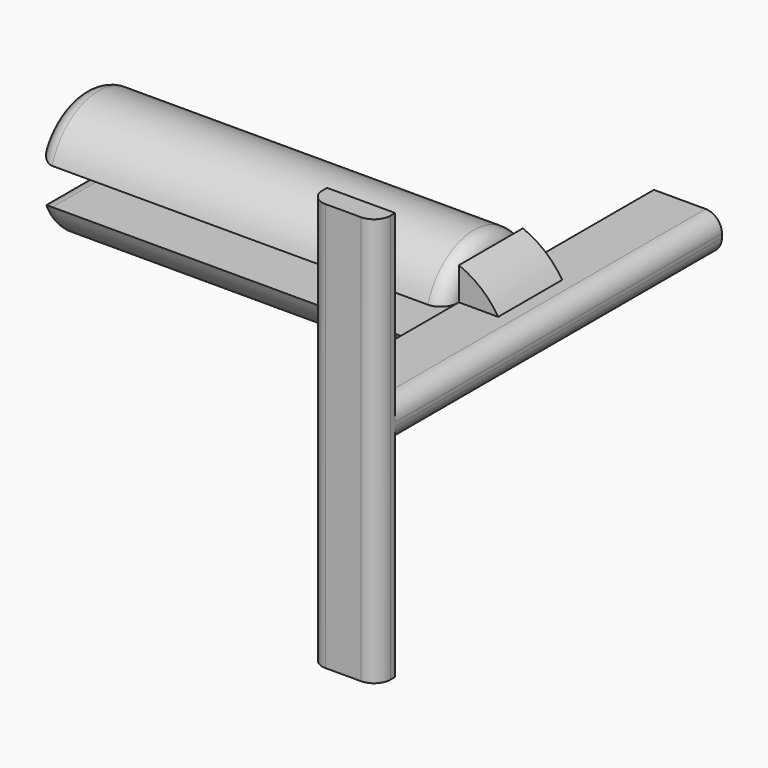
from build123d import *

# Parameters (mm, degrees)
F0_W        = 4.1652182117
F0_H        = 1.361677656
F1_DEPTH    = 25
F2_W        = 4.1652182117
F2_H        = 2.2310467437
F3_DEPTH    = 25
F5_DEPTH    = 25
F6_R        = 1
F6_2_R      = 1
F6_3_R      = 1
F7_W        = 3.1652182117
F7_H        = 4.8921946436
F8_DEPTH    = 2
F9_T1_DEPTH = 28.1481486067


# Not quite as in the source:
# - a fillet or chamfer that OpenCascade refuses, or shapes differently, is made with other operations: its cross-section is extruded or revolved along the edge and cut away or added


with BuildPart() as f1:
    # F0 (on Top) → F1 (new body)
    with BuildSketch(Plane.XY):
        with Locations((-2.0826091059, 0.680838828)):
            Rectangle(F0_W, F0_H)
    extrude(amount=F1_DEPTH)

    # F2 (on face) → F3 (join)
    with BuildSketch(Plane(origin=(0, 1.361677656, 0), x_dir=(-1, 0, 0), z_dir=(0, 1, 0))):
        with Locations((2.0826091059, 13.6155233718)):
            Rectangle(F2_W, F2_H)
    extrude(amount=F3_DEPTH)

    # F6
    f6_edges = [f1.edges().sort_by_distance(p)[0] for p in [
        (-4.165218, 0, 12.5),
        (0, 0, 12.5),
        (0, 13.861678, 14.731047),
        (0, 13.861678, 12.5),
    ]]
    fillet(f6_edges, radius=F6_R)


with BuildPart() as f5:
    # F4 (on face) → F5 (new body)
    with BuildSketch(Plane(origin=(-4.1652182117, 0, 0), x_dir=(0, -1, 0), z_dir=(-1, 0, 0))):
        with BuildLine():
            Line((-17.3905032205, 14.7310467437), (-10.3328520914, 14.7310467437))
            ThreePointArc((-10.3328520914, 14.7310467437), (-13.861677656, 17.3342168413), (-17.3905032205, 14.7310467437))
        make_face()
    extrude(amount=F5_DEPTH)

    # F6#2
    f6_2_edges = [f5.edges().sort_by_distance(p)[0] for p in [
        (-4.165218, 13.861678, 17.334217),
        (-29.165218, 13.861678, 14.731047),
        (-29.165218, 13.861678, 17.334217),
    ]]
    fillet(f6_2_edges, radius=F6_2_R)


with BuildPart() as f5b:
    # F4 (on face) → F5, piece 2 (new body)
    with BuildSketch(Plane(origin=(-4.1652182117, 0, 0), x_dir=(0, -1, 0), z_dir=(-1, 0, 0))):
        with BuildLine():
            ThreePointArc((-17.3744763274, 12.5), (-13.861677656, 9.947413943), (-10.3488789845, 12.5))
            Line((-10.3488789845, 12.5), (-17.3744763274, 12.5))
        make_face()
    extrude(amount=F5_DEPTH)

    # F6#3
    f6_3_edges = [f5b.edges().sort_by_distance(p)[0] for p in [
        (-4.165218, 13.861678, 9.947414),
        (-29.165218, 13.861678, 9.947414),
        (-29.165218, 13.861678, 12.5),
    ]]
    fillet(f6_3_edges, radius=F6_3_R)


with BuildPart() as f8:
    # F7 (on face) → F8 (new body)
    with BuildSketch(Plane.XY.offset(14.7310467437)):
        with Locations((-2.5826091059, 13.8936350122)):
            Rectangle(F7_W, F7_H)
    extrude(amount=F8_DEPTH)

    # F9: fillet of radius 5 on 1 edges, made by hand

    # F9_s2 → F9_t1 (cut)
    with BuildSketch(Plane.XZ.offset(-27.9677093156)):
        with BuildLine():
            ThreePointArc((-1, 12.0798559511), (-1.8663630456, 14.8928695538), (-4.1652182117, 16.7310467437))
            Line((-4.1652182117, 16.7310467437), (-4.1285225759, 16.8240705595))
            ThreePointArc((-4.1285225759, 16.8240705595), (-2.5826091059, 16.8310467437), (-1, 16.8310467437))
            Line((-1, 16.8310467437), (-0.9, 16.7310467437))
            Line((-0.9, 16.7310467437), (-0.9, 12.0798559511))
            Line((-0.9, 12.0798559511), (-1, 12.0798559511))
        make_face()
    extrude(amount=F9_T1_DEPTH, mode=Mode.SUBTRACT)


solid = Compound([f1.part, f5.part, f5b.part, f8.part])
